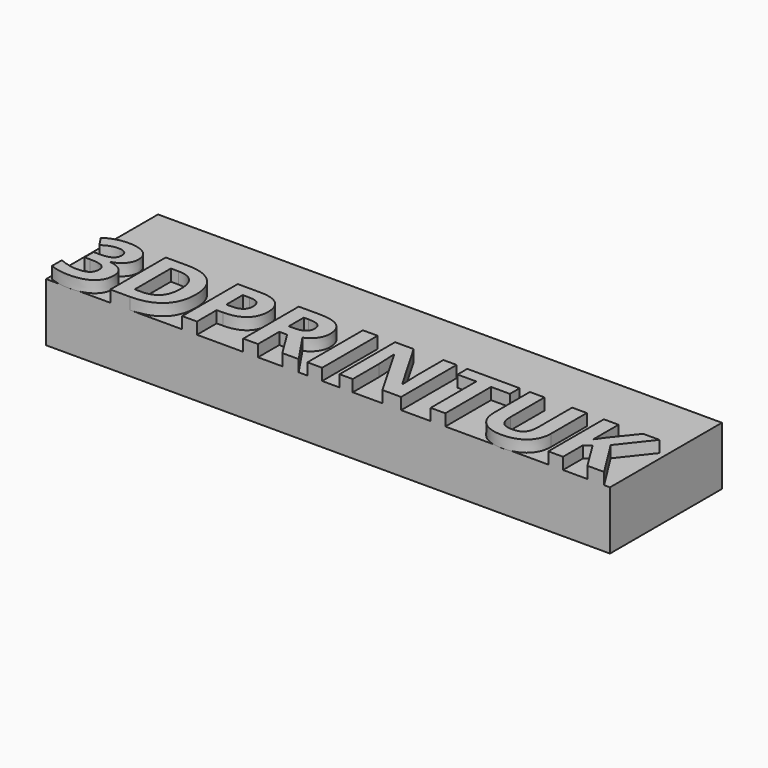
from build123d import *

# Parameters (mm, degrees)
F0_W         = 56.7791811411
F0_H         = 60
F1_DEPTH     = 25
F3_DEPTH     = 185
F2_TEXT_SIZE = 41.6666666667
F4_DEPTH     = 5


# Not quite as in the source:
# - Text() gives the source's letters only with a copy of the font that has no kerning and outlines rounded to 1/6400 em; it was checked with that copy


with BuildPart() as f1:
    # F0 (on Top) → F1 (new body)
    with BuildSketch(Plane.XY):
        Rectangle(F0_W, F0_H)
    extrude(amount=F1_DEPTH)

    # F3 (add): a face of the model
    f3_faces = [f1.faces().sort_by_distance(p)[0] for p in [
        (28.3895905706, 0, 12.5),
    ]]
    extrude(f3_faces, amount=F3_DEPTH)

    # F2 (on face) → F4 (join)
    with BuildSketch(Plane.XY.offset(25)):
        with Locations((-28.3895905706, -30)):
            Text('3DPRINTUK', F2_TEXT_SIZE, font='Open Sans', font_style=FontStyle.BOLD, text_align=(TextAlign.LEFT, TextAlign.BOTTOM))
    extrude(amount=F4_DEPTH)


solid = f1.part
